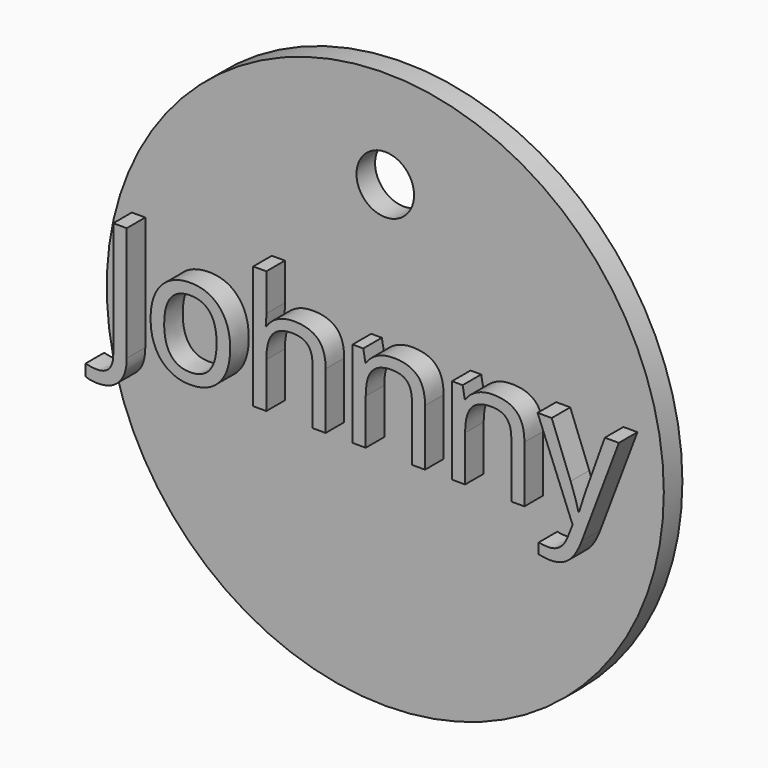
from build123d import *

# Parameters (mm, degrees)
F0_R         = 60
F1_DEPTH     = 5
F2_TEXT_SIZE = 34.8781304909
F3_DEPTH     = 5
F4_R         = 6.1981825103
F5_DEPTH     = 10


# Not quite as in the source:
# - Text() gives the source's letters only with a copy of the font that has no kerning and outlines rounded to 1/6400 em; it was checked with that copy


with BuildPart() as f1:
    # F0 (on Front) → F1 (new body)
    with BuildSketch(Plane.XZ):
        Circle(F0_R)
    extrude(amount=F1_DEPTH)

    # F2 (on face) → F3 (join)
    with BuildSketch(Plane.XZ.offset(5)):
        with Locations((-57.8255811205, -9.1059374477)):
            Text('Johnny', F2_TEXT_SIZE, font='Open Sans', text_align=(TextAlign.LEFT, TextAlign.BOTTOM))
    extrude(amount=F3_DEPTH)

    # F4 (on face) → F5 (cut)
    with BuildSketch(Plane.XZ.offset(5)):
        with Locations((0, 38.8437062502)):
            Circle(F4_R)
    extrude(amount=-F5_DEPTH, mode=Mode.SUBTRACT)


solid = f1.part
